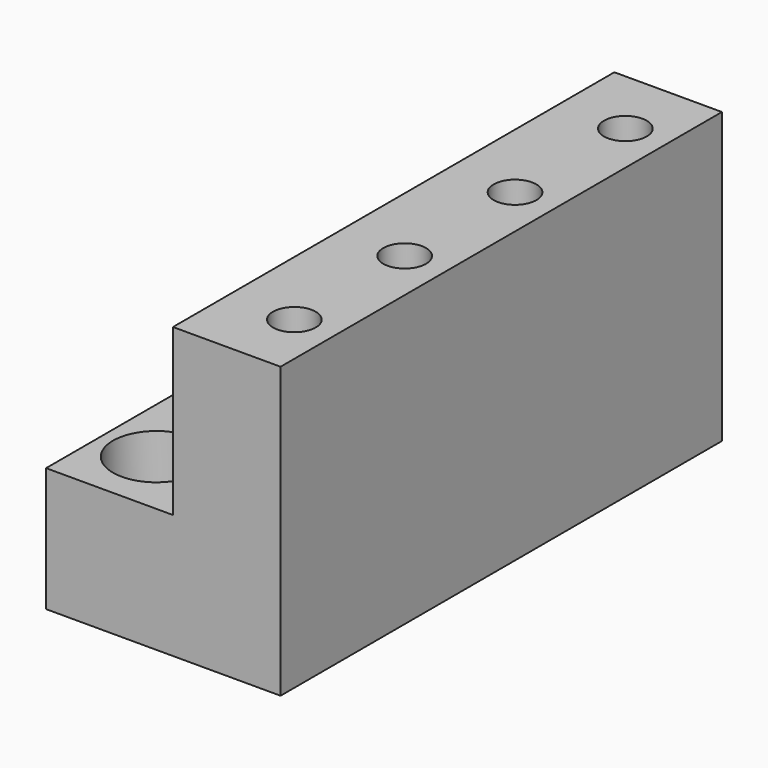
from build123d import *

# Parameters (mm, degrees)
F0_W           = 39
F0_H           = 60
F1_DEPTH       = 200
F4_D           = 15.5
F4_DEPTH       = 18
F4_TIP         = 4.6566697975
F5_D           = 22
F5_CBORE_D     = 31.5
F5_CBORE_DEPTH = 20


# Not quite as in the source:
# - a feature names something its author has since deleted; it is built from what else it names


with BuildPart() as f1:
    # F0 (on Front) → F1 (new body)
    with BuildSketch(Plane.XZ):
        with Locations((19.5, 75)):
            Rectangle(F0_W, F0_H)
        Polygon((0, 45), (-46, 45), (-46, 0), (39, 0), (39, 45), align=None)
    extrude(amount=-F1_DEPTH)

    # F4
    with Locations(Plane.XY.offset(105)):
        with Locations((24, 25), (24, 75), (24, 125), (24, 175)):
            Hole(F4_D / 2, depth=F4_DEPTH)
            with Locations((0, 0, -(F4_DEPTH + F4_TIP / 2))):  # 118° drill point
                Cone(0, F4_D / 2, F4_TIP, mode=Mode.SUBTRACT)

    # F5 (through all)
    with Locations(Plane.XY.offset(45)):
        with Locations((-26, 25), (-26, 75), (-26, 125), (-26, 175)):
            CounterBoreHole(F5_D / 2, F5_CBORE_D / 2, F5_CBORE_DEPTH)


solid = f1.part
